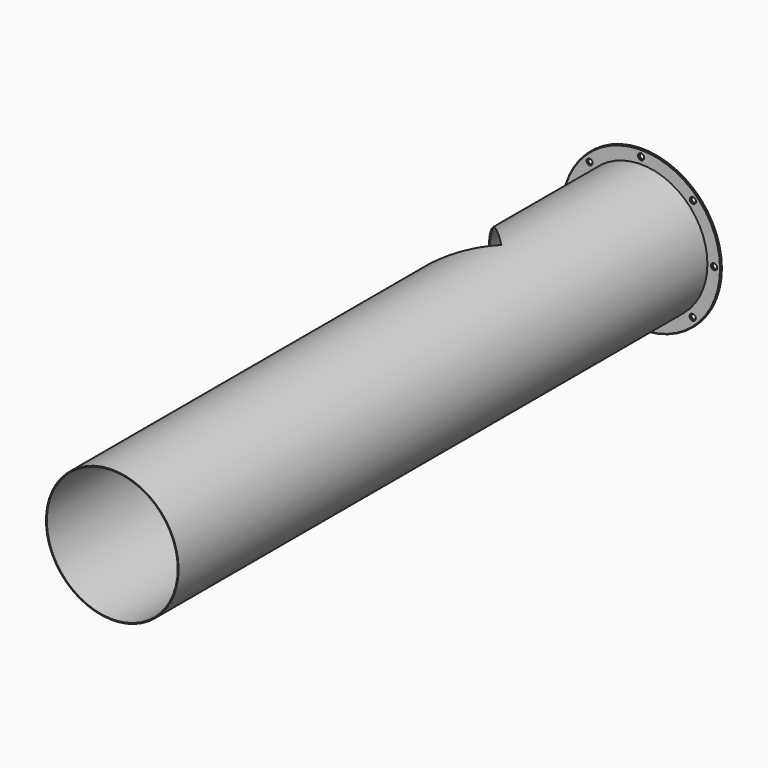
from build123d import *

# Parameters (mm, degrees)
F0_R     = 150
F0_R_2   = 148
F1_DEPTH = 1500
F0_R_3   = 180
F0_R_4   = 5.5
F2_DEPTH = 5
F3_R     = 1.99999
F4_SIZE  = 1.5
F5_R     = 150
F6_DEPTH = 180.001


# Not quite as in the source:
# - a fillet or chamfer is up to 0.001 mm smaller than in the source, because OpenCascade refuses the exact size


with BuildPart() as f1:
    # F0 (on Front) → F1 (new body)
    with BuildSketch(Plane.XZ):
        Circle(F0_R)
        Circle(F0_R_2, mode=Mode.SUBTRACT)
    extrude(amount=F1_DEPTH)

    # F3 (radius 2 in the source; OpenCascade refuses exactly that, so slightly less here)
    f3_edges = [f1.edges().sort_by_distance(p)[0] for p in [
        (-148, 0, 0),
    ]]
    fillet(f3_edges, radius=F3_R)

    # F5 (on Right) → F6 (cut, through all)
    with BuildSketch(Plane.YZ):
        with Locations((-400, 0)):
            Circle(F5_R)
    extrude(amount=-F6_DEPTH, mode=Mode.SUBTRACT)


with BuildPart() as f2:
    # F0 (on Front) → F2 (new body)
    with BuildSketch(Plane.XZ):
        Circle(F0_R_3)
        with Locations((-116.1570210146, -117.1859482576)):
            Circle(F0_R_4, mode=Mode.SUBTRACT)
        with Locations((0, -165)):
            Circle(F0_R_4, mode=Mode.SUBTRACT)
        with Locations((116.7257672626, -116.619446307)):
            Circle(F0_R_4, mode=Mode.SUBTRACT)
        with Locations((-165, 0)):
            Circle(F0_R_4, mode=Mode.SUBTRACT)
        with Locations((-116.619446307, 116.7257672626)):
            Circle(F0_R_4, mode=Mode.SUBTRACT)
        Circle(F0_R, mode=Mode.SUBTRACT)
        with Locations((165, 0)):
            Circle(F0_R_4, mode=Mode.SUBTRACT)
        with Locations((0, 165)):
            Circle(F0_R_4, mode=Mode.SUBTRACT)
        with Locations((117.1859482576, 116.1570210146)):
            Circle(F0_R_4, mode=Mode.SUBTRACT)
    extrude(amount=F2_DEPTH)

    # F4
    f4_edges = [f2.edges().sort_by_distance(p)[0] for p in [
        (-180, -5, 0),
        (-180, 0, 0),
        (159.5, 0, 0),
        (111.685948, 0, 116.157021),
        (111.685948, -5, 116.157021),
        (159.5, -5, 0),
        (111.225767, -5, -116.619446),
        (-121.657021, -5, -117.185948),
        (-170.5, -5, 0),
        (-122.119446, -5, 116.725767),
        (-5.5, -5, 165),
        (-121.657021, 0, -117.185948),
        (-170.5, 0, 0),
        (-122.119446, 0, 116.725767),
        (-5.5, 0, 165),
        (-5.5, 0, -165),
        (111.225767, 0, -116.619446),
        (-5.5, -5, -165),
    ]]
    chamfer(f4_edges, length=F4_SIZE)


solid = Compound([f1.part, f2.part])
